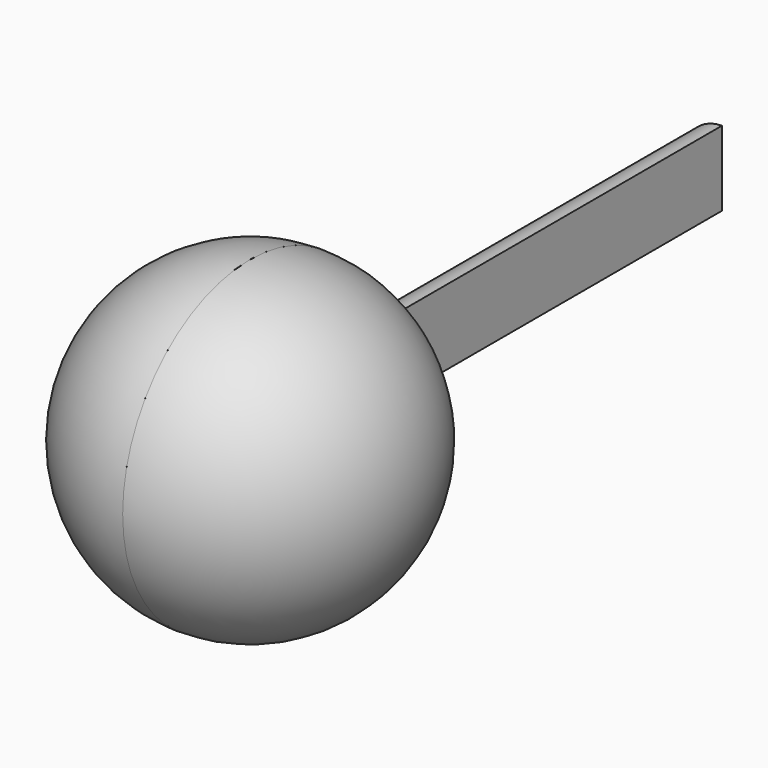
from build123d import *
from build123d import SkipClean  # not in build123d's __all__

# Parameters (mm, degrees)
F1_ANGLE_START = 90
F1_ANGLE       = 180
F5_START       = -25.4
F5_DEPTH       = 68.58
F7_ANGLE_BACK  = 180
F7_ANGLE       = 180
F8_R           = 6.35
F9_DEPTH       = 25.654
F10_DEPTH      = 24.892


with BuildPart() as f1:
    # F0 (on Front) → F1 (revolve)
    with BuildSketch(Plane.XZ, mode=Mode.PRIVATE) as f1_sk:
        with BuildLine():
            ThreePointArc((25.2817304641, 2.448286082), (17.0729835342, 18.8062019887), (0, 25.4))
            Line((0, 25.4), (0, -25.4))
            ThreePointArc((0, -25.4), (18.8062019887, -17.0729835342), (25.2817304641, 2.448286082))
        make_face()
    revolve(f1_sk.sketch.rotate(Axis((0, 0, 0), (0, 0, 1)), F1_ANGLE_START), axis=Axis((0, 0, 0), (0, 0, 1)), revolution_arc=F1_ANGLE)

    # F2 (on Front) → F3 (revolve, cut)
    with BuildSketch(Plane.XZ):
        with BuildLine():
            Line((0, -22.86), (0, 22.86))
            ThreePointArc((0, 22.86), (-22.86, 0), (0, -22.86))
        make_face()
    with SkipClean():  # cleaning this boolean's faces spoils the solid; the shape is the same uncleaned
        revolve(axis=Axis((0, 0, 0), (0, 0, -1)), mode=Mode.SUBTRACT)


with BuildPart() as f5:
    # F4 (on Front) → F5 (new body)
    with BuildSketch(Plane.XZ.offset(F5_START)):
        with BuildLine():
            ThreePointArc((0, 5.969), (-5.969, 0), (0, -5.969))
            Line((0, -5.969), (0, 5.969))
        make_face()
    extrude(amount=-F5_DEPTH)


with BuildPart() as f7:
    # F6 (on Right) → F7 (revolve)
    with BuildSketch(Plane.YZ, mode=Mode.PRIVATE) as f7_sk:
        with BuildLine():
            ThreePointArc((-22.86, 0), (0, 22.86), (22.86, 0))
            Line((22.86, 0), (25.4, 0))
            ThreePointArc((25.4, 0), (0, 25.4), (-25.4, 0))
            Line((-25.4, 0), (-22.86, 0))
        make_face()
    revolve(f7_sk.sketch.rotate(Axis((0, 0, 0), (0, -1, 0)), -F7_ANGLE_BACK), axis=Axis((0, 0, 0), (0, -1, 0)), revolution_arc=F7_ANGLE)


with BuildPart() as f9_tool:
    # F8 (on Front) → F9 (new body)
    with BuildSketch(Plane.XZ):
        Circle(F8_R)
    extrude(amount=-F9_DEPTH)


with BuildPart() as f1_1:
    add(f1.part, clean=False)

    # F9: cut by f9_tool
    add(f9_tool.part, mode=Mode.SUBTRACT)

    # F8 (on Front) → F10 (cut)
    with BuildSketch(Plane.XZ):
        Circle(F8_R)
    extrude(amount=-F10_DEPTH, mode=Mode.SUBTRACT)


with BuildPart() as f7_1:
    add(f7.part, clean=False)

    # F9: cut by f9_tool
    add(f9_tool.part, mode=Mode.SUBTRACT)


solid = Compound([f5.part, f1_1.part, f7_1.part])
